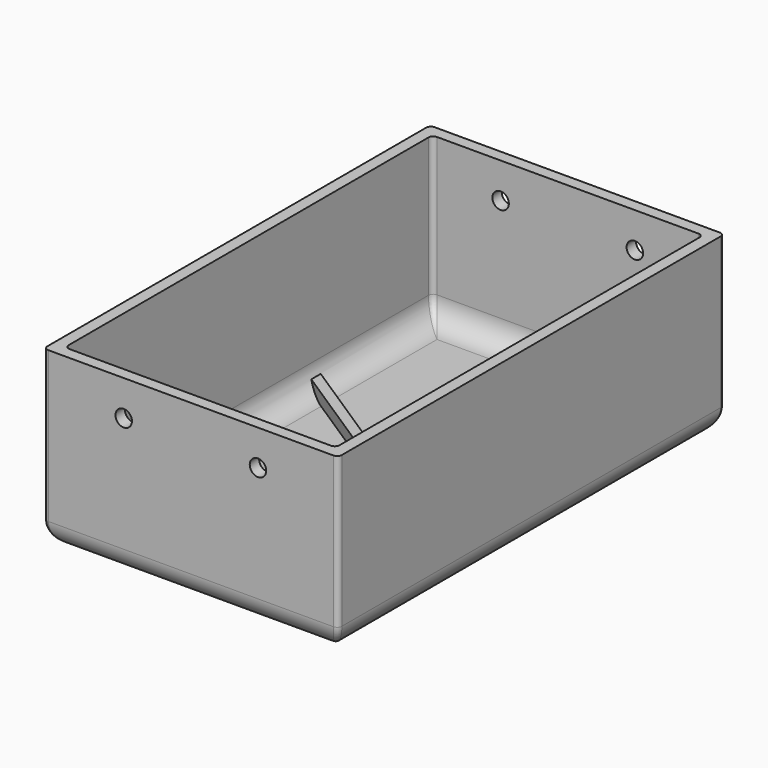
from build123d import *

# Parameters (mm, degrees)
F1_W          = 62.5
F1_H          = 102.5
F1_W_2        = 57.5
F1_H_2        = 97.5
F2_DEPTH      = 37
F3_W          = 62.5
F3_H          = 102.5
F4_DEPTH      = 2.5
F6_DEPTH      = 2.501
F7_W          = 51
F7_H          = 72
F8_DEPTH      = 1.2
F10_DEPTH     = 2.5
F11_R         = 1.75
F12_DEPTH     = 102.501
F13_T1_DEPTH  = 42.5
F13_T3_DEPTH  = 57.5
F13_T5_DEPTH  = 42.5
F13_T7_DEPTH  = 57.5
F13_T9_DEPTH  = 44.4614347816
F13_T11_DEPTH = 57.9568101466
F13_T13_DEPTH = 40.0817550719
F13_T15_DEPTH = 127.5
F13_T17_DEPTH = 87.5
F14_R         = 1


# Not quite as in the source:
# - a fillet or chamfer that OpenCascade refuses, or shapes differently, is made with other operations: its cross-section is extruded or revolved along the edge and cut away or added


with BuildPart() as f2:
    # F1 (on Top) → F2 (new body)
    with BuildSketch(Plane.XY):
        with Locations((28.75, 48.75)):
            Rectangle(F1_W, F1_H)
        with Locations((28.75, 48.75)):
            Rectangle(F1_W_2, F1_H_2, mode=Mode.SUBTRACT)
    extrude(amount=F2_DEPTH)

    # F3 (on Top) → F4 (join)
    with BuildSketch(Plane.XY):
        with Locations((28.75, 48.75)):
            Rectangle(F3_W, F3_H)
    extrude(amount=F4_DEPTH)

    # F5 (on face) → F6 (cut, through all)
    with BuildSketch(Plane.XY.offset(2.5)):
        with BuildLine():
            ThreePointArc((17.25, 90.5), (16.25, 89.5), (17.25, 88.5))
            Line((17.25, 88.5), (40.25, 88.5))
            ThreePointArc((40.25, 88.5), (41.25, 89.5), (40.25, 90.5))
            Line((40.25, 90.5), (17.25, 90.5))
        make_face()
        with BuildLine():
            ThreePointArc((17.25, 13), (16.25, 12), (17.25, 11))
            Line((17.25, 11), (40.25, 11))
            ThreePointArc((40.25, 11), (41.25, 12), (40.25, 13))
            Line((40.25, 13), (17.25, 13))
        make_face()
    extrude(amount=-F6_DEPTH, mode=Mode.SUBTRACT)

    # F7 (on face) → F8 (cut)
    with BuildSketch(Plane(origin=(0, 0, 0), x_dir=(1, 0, 0), z_dir=(0, 0, -1))):
        with Locations((28.75, -53.5)):
            Rectangle(F7_W, F7_H)
    extrude(amount=-F8_DEPTH, mode=Mode.SUBTRACT)

    # F9 (on face) → F10 (join)
    with BuildSketch(Plane.XY.offset(2.5)):
        Polygon((0, 32.5), (0, 30), (28.5635979803, 46.412179039), (26.5233409817, 47.7398805363), align=None)
        Polygon((26.5233409817, 47.7398805363), (28.5635979803, 46.412179039), (30.6038549789, 47.5844775418), (28.5635979803, 48.912179039), align=None)
        Polygon((30.6038549789, 47.5844775418), (28.5635979803, 46.412179039), (57.5, 27.5817550719), (57.5, 30.0817550719), align=None)
        Polygon((28.5635979803, 48.912179039), (30.6038549789, 47.5844775418), (57.5, 63.0385652184), (57.5, 65.5385652184), align=None)
        Polygon((0, 65), (26.5233409817, 47.7398805363), (28.5635979803, 48.912179039), (0, 67.5), align=None)
    extrude(amount=F10_DEPTH)

    # F11 (on face) → F12 (cut, through all)
    with BuildSketch(Plane(origin=(0, 100, 0), x_dir=(-1, 0, 0), z_dir=(0, 1, 0))):
        with Locations((-14.5, 29.5)):
            Circle(F11_R)
        with Locations((-43, 29.5)):
            Circle(F11_R)
    extrude(amount=-F12_DEPTH, mode=Mode.SUBTRACT)

    # F13: fillet of radius 5 on 12 edges, made by hand

    # F13_s2 → F13_t1 (join)
    with BuildSketch(Plane.XZ.offset(-42.5)):
        with BuildLine():
            ThreePointArc((0, 7.5), (1.4644660941, 3.9644660941), (5, 2.5))
            Line((5, 2.5), (0, 2.5))
            Line((0, 2.5), (0, 7.5))
        make_face()
    extrude(amount=F13_T1_DEPTH)

    # F13_s4 → F13_t3 (join)
    with BuildSketch(Plane.XZ.offset(-77.5)):
        with BuildLine():
            ThreePointArc((0, 7.5), (1.4644660941, 3.9644660941), (5, 2.5))
            Line((5, 2.5), (0, 2.5))
            Line((0, 2.5), (0, 7.5))
        make_face()
    extrude(amount=F13_T3_DEPTH)

    # F13_s6 → F13_t5 (join)
    with BuildSketch(Plane.XZ.offset(-97.5)):
        with BuildLine():
            ThreePointArc((0, 7.5), (1.4644660941, 3.9644660941), (5, 2.5))
            Line((5, 2.5), (0, 2.5))
            Line((0, 2.5), (0, 7.5))
        make_face()
    extrude(amount=F13_T5_DEPTH)

    # F13_s8 → F13_t7 (join)
    with BuildSketch(Plane.YZ):
        with BuildLine():
            ThreePointArc((0, 7.5), (1.4644660941, 3.9644660941), (5, 2.5))
            Line((5, 2.5), (0, 2.5))
            Line((0, 2.5), (0, 7.5))
        make_face()
        with BuildLine():
            ThreePointArc((97.5, 7.5), (96.0355339059, 3.9644660941), (92.5, 2.5))
            Line((92.5, 2.5), (97.5, 2.5))
            Line((97.5, 2.5), (97.5, 7.5))
        make_face()
    extrude(amount=F13_T7_DEPTH)

    # F13_s10 → F13_t9 (join)
    with BuildSketch(Plane.XZ.offset(-97.5)):
        with BuildLine():
            ThreePointArc((57.5, 7.5), (56.0355339059, 3.9644660941), (52.5, 2.5))
            Line((52.5, 2.5), (57.5, 2.5))
            Line((57.5, 2.5), (57.5, 7.5))
        make_face()
    extrude(amount=F13_T9_DEPTH)

    # F13_s12 → F13_t11 (join)
    with BuildSketch(Plane.XZ.offset(-75.5385652184)):
        with BuildLine():
            ThreePointArc((57.5, 7.5), (56.0355339059, 3.9644660941), (52.5, 2.5))
            Line((52.5, 2.5), (57.5, 2.5))
            Line((57.5, 2.5), (57.5, 7.5))
        make_face()
    extrude(amount=F13_T11_DEPTH)

    # F13_s14 → F13_t13 (join)
    with BuildSketch(Plane.XZ.offset(-40.0817550719)):
        with BuildLine():
            ThreePointArc((57.5, 7.5), (56.0355339059, 3.9644660941), (52.5, 2.5))
            Line((52.5, 2.5), (57.5, 2.5))
            Line((57.5, 2.5), (57.5, 7.5))
        make_face()
    extrude(amount=F13_T13_DEPTH)

    # F13_s16 → F13_t15 (cut)
    with BuildSketch(Plane.XZ.offset(-112.5)):
        with BuildLine():
            ThreePointArc((-2.5, 5), (-1.0355339059, 1.4644660941), (2.5, 0))
            Line((2.5, 0), (-2.5, 0))
            Line((-2.5, 0), (-2.5, 5))
        make_face()
        with BuildLine():
            ThreePointArc((60, 5), (58.5355339059, 1.4644660941), (55, 0))
            Line((55, 0), (60, 0))
            Line((60, 0), (60, 5))
        make_face()
    extrude(amount=F13_T15_DEPTH, mode=Mode.SUBTRACT)

    # F13_s18 → F13_t17 (cut)
    with BuildSketch(Plane.YZ.offset(-15)):
        with BuildLine():
            ThreePointArc((100, 5), (98.5355339059, 1.4644660941), (95, 0))
            Line((95, 0), (100, 0))
            Line((100, 0), (100, 5))
        make_face()
        with BuildLine():
            ThreePointArc((-2.5, 5), (-1.0355339059, 1.4644660941), (2.5, 0))
            Line((2.5, 0), (-2.5, 0))
            Line((-2.5, 0), (-2.5, 5))
        make_face()
    extrude(amount=F13_T17_DEPTH, mode=Mode.SUBTRACT)

    # F14
    f14_edges = [f2.edges().sort_by_distance(p)[0] for p in [
        (60, 100, 21),
        (-2.5, 100, 21),
        (-2.5, -2.5, 21),
        (60, -2.5, 21),
        (0, 0, 22.25),
        (57.5, 0, 22.25),
        (57.5, 97.5, 22.25),
        (0, 97.5, 22.25),
        (-1.035534, 98.535534, 1.464466),
        (58.535534, 98.535534, 1.464466),
        (-1.035534, -1.035534, 1.464466),
        (58.535534, -1.035534, 1.464466),
        (56.035534, 1.464466, 3.964466),
        (1.464466, 1.464466, 3.964466),
        (1.464466, 96.035534, 3.964466),
        (56.035534, 96.035534, 3.964466),
    ]]
    fillet(f14_edges, radius=F14_R)


solid = f2.part
